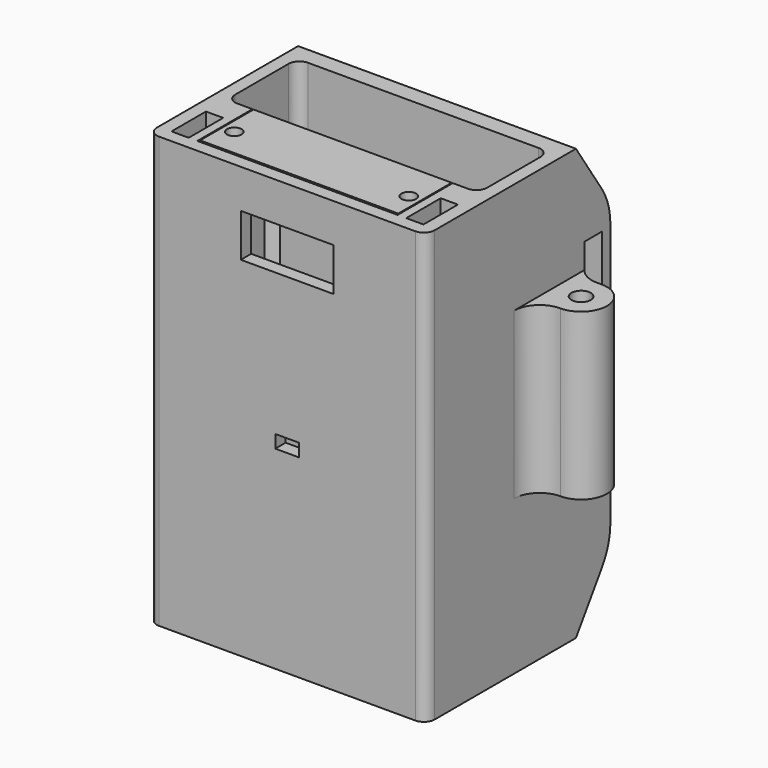
from build123d import *

# Parameters (mm, degrees)
F0_W         = 4
F0_H         = 10
F1_DEPTH     = 100
F2_START     = -3
F0_R         = 1.5
F2_DEPTH     = 97
F3_START     = -28
F3_DEPTH     = 72
F4_START     = -95
F4_DEPTH     = 5
F5_START     = -66
F0_W_2       = 34.5
F0_H_2       = 14
F5_DEPTH     = 34
F6_START     = -25.8
F0_R_2       = 3.75
F0_R_3       = 2.25
F6_DEPTH     = 38.4
F7_START     = -82
F7_DEPTH     = 18
F8_W         = 5
F8_H         = 50
F9_DEPTH     = 64.5
F10_W        = 46
F10_H        = 15.5
F10_R        = 1.7
F11_DEPTH    = 3
F12_W        = 21.5
F12_H        = 10
F12_W_2      = 5.5
F12_H_2      = 3
F13_DEPTH    = 3
F14_R        = 2.5
F15_R        = 2.5
F16_T1_DEPTH = 38.4
F17_R        = 15
F18_SIZE     = 2


# Not quite as in the source:
# - a fillet or chamfer that OpenCascade refuses, or shapes differently, is made with other operations: its cross-section is extruded or revolved along the edge and cut away or added


with BuildPart() as f1:
    # F0 (on Top) → F1 (new body)
    with BuildSketch(Plane.XY):
        Polygon((64.5, 43.5), (0, 43.5), (0, 31.5), (0, 0), (64.5, 0), (64.5, 31.5), align=None)
        with Locations((5, 8)):
            Rectangle(F0_W, F0_H, mode=Mode.SUBTRACT)
        with Locations((59.5, 8)):
            Rectangle(F0_W, F0_H, mode=Mode.SUBTRACT)
        Polygon((9, 19), (3, 19), (3, 39.5), (61.5, 39.5), (61.5, 19), (55.5, 19), (55.5, 3), (49.5, 3), (15, 3), (9, 3), align=None, mode=Mode.SUBTRACT)
    extrude(amount=-F1_DEPTH)

    # F0 (on Top) → F2 (join)
    with BuildSketch(Plane.XY.offset(F2_START)):
        Polygon((55.5, 19), (9, 19), (9, 3), (15, 3), (15, 17), (49.5, 17), (49.5, 3), (55.5, 3), align=None)
        with Locations((12, 10)):
            Circle(F0_R, mode=Mode.SUBTRACT)
        with Locations((52.5, 10)):
            Circle(F0_R, mode=Mode.SUBTRACT)
    extrude(amount=-F2_DEPTH)

    # F0 (on Top) → F3 (join)
    with BuildSketch(Plane.XY.offset(F3_START)):
        with Locations((52.5, 10)):
            Circle(F0_R)
        with Locations((12, 10)):
            Circle(F0_R)
    extrude(amount=-F3_DEPTH)

    # F0 (on Top) → F4 (join)
    with BuildSketch(Plane.XY.offset(F4_START)):
        Polygon((3, 39.5), (3, 19), (9, 19), (55.5, 19), (61.5, 19), (61.5, 39.5), align=None)
    extrude(amount=-F4_DEPTH)

    # F0 (on Top) → F5 (join)
    with BuildSketch(Plane.XY.offset(F5_START)):
        with Locations((32.25, 10)):
            Rectangle(F0_W_2, F0_H_2)
    extrude(amount=-F5_DEPTH)

    # F0 (on Top) → F6 (join)
    with BuildSketch(Plane.XY.offset(F6_START)):
        with BuildLine():
            Line((70.5, 43.5), (64.5, 43.5))
            Line((64.5, 43.5), (64.5, 31.5))
            Line((64.5, 31.5), (70.5, 31.5))
            ThreePointArc((70.5, 31.5), (76.5, 37.5), (70.5, 43.5))
        make_face()
        with Locations((70.5, 37.5)):
            Circle(F0_R_2, mode=Mode.SUBTRACT)
        with Locations((70.5, 37.5)):
            Circle(F0_R_2)
        with Locations((70.5, 37.5)):
            Circle(F0_R_3, mode=Mode.SUBTRACT)
    extrude(amount=-F6_DEPTH)

    # F0 (on Top) → F7 (join)
    with BuildSketch(Plane.XY.offset(F7_START)):
        with Locations((5, 8)):
            Rectangle(F0_W, F0_H)
        with Locations((59.5, 8)):
            Rectangle(F0_W, F0_H)
    extrude(amount=-F7_DEPTH)

    # F8 (on face) → F9 (join, through all)
    with BuildSketch(Plane.YZ.offset(64.5)):
        Polygon((53.5, -15), (43.5, 0), (43.5, -25.8), (31.5, -25.8), (31.5, -64.2), (43.5, -64.2), (43.5, -100), (53.5, -85), align=None)
        with Locations((48.5, -45)):
            Rectangle(F8_W, F8_H, mode=Mode.SUBTRACT)
    extrude(amount=-F9_DEPTH)

    # F12 (on face) → F13 (cut, through all)
    with BuildSketch(Plane(origin=(0, 3, 0), x_dir=(-1, 0, 0), z_dir=(0, 1, 0))):
        with Locations((-32.25, -14)):
            Rectangle(F12_W, F12_H)
        with Locations((-32.25, -53.5)):
            Rectangle(F12_W_2, F12_H_2)
    extrude(amount=-F13_DEPTH, mode=Mode.SUBTRACT)

    # F14
    f14_edges = [f1.edges().sort_by_distance(p)[0] for p in [
        (3, 39.5, -12.9),
        (3, 39.5, -79.6),
        (61.5, 39.5, -12.9),
        (61.5, 39.5, -79.6),
        (61.5, 19, -47.5),
        (3, 19, -47.5),
    ]]
    fillet(f14_edges, radius=F14_R)

    # F15
    f15_edges = [f1.edges().sort_by_distance(p)[0] for p in [
        (0, 0, -50),
        (64.5, 0, -50),
    ]]
    fillet(f15_edges, radius=F15_R)

    # F16: fillet of radius 6 on 2 edges, made by hand

    # F16_s2 → F16_t1 (join)
    with BuildSketch(Plane.XY.offset(-64.2)):
        with BuildLine():
            ThreePointArc((64.5, 25.5), (66.2573593129, 29.7426406871), (70.5, 31.5))
            Line((70.5, 31.5), (64.5, 31.5))
            Line((64.5, 31.5), (64.5, 25.5))
        make_face()
        with BuildLine():
            ThreePointArc((64.5, 46), (66.6347843849, 44.161460874), (69.3733971724, 43.5))
            Line((69.3733971724, 43.5), (64.5, 43.5))
            Line((64.5, 43.5), (64.5, 46))
        make_face()
    extrude(amount=F16_T1_DEPTH)

    # F17
    f17_edges = [f1.edges().sort_by_distance(p)[0] for p in [
        (32.25, 53.5, -15),
        (32.25, 53.5, -85),
    ]]
    fillet(f17_edges, radius=F17_R)

    # F18
    f18_edges = [f1.edges().sort_by_distance(p)[0] for p in [
        (15, 17, -34.5),
        (49.5, 17, -34.5),
    ]]
    chamfer(f18_edges, length=F18_SIZE)


with BuildPart() as f11:
    # F10 (on face) → F11 (new body, through all)
    with BuildSketch(Plane.XY.offset(-3)):
        with Locations((32.25, 11.25)):
            Rectangle(F10_W, F10_H)
        with Locations((12, 10)):
            Circle(F10_R, mode=Mode.SUBTRACT)
        with Locations((52.5, 10)):
            Circle(F10_R, mode=Mode.SUBTRACT)
    extrude(amount=F11_DEPTH)


solid = Compound([f1.part, f11.part])
